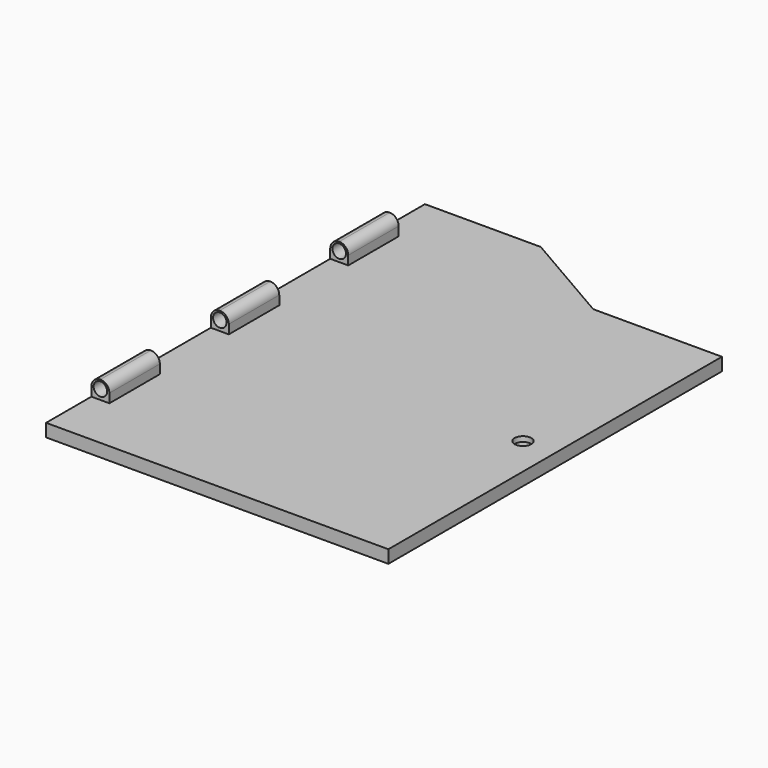
from build123d import *

# Parameters (mm, degrees)
F0_W     = 7
F0_H     = 24.5
F1_DEPTH = 5
F2_W     = 7
F2_H     = 24.5
F3_DEPTH = 7
F4_R     = 3.49999
F5_R     = 2.625
F6_DEPTH = 162.001
F7_R     = 3.25
F8_DEPTH = 2


# Not quite as in the source:
# - a fillet or chamfer is up to 0.001 mm smaller than in the source, because OpenCascade refuses the exact size


with BuildPart() as f1:
    # F0 (on Top) → F1 (new body)
    with BuildSketch(Plane.XY):
        Polygon((-34.0007612563, 142.7090217992), (-79.0007612563, 142.7090217992), (-79.0007612563, 121.2090217992), (-72.0007612563, 121.2090217992), (-72.0007612563, 96.7090217992), (-79.0007612563, 96.7090217992), (-79.0007612563, 63.2090217992), (-72.0007612563, 63.2090217992), (-72.0007612563, 38.7090217992), (-79.0007612563, 38.7090217992), (-79.0007612563, 5.2090217992), (-72.0007612563, 5.2090217992), (-72.0007612563, -19.2909782008), (-79.0007612563, -19.2909782008), (-79.0007612563, -41.2909782008), (53.9992387437, -41.2909782008), (53.9992387437, 120.7090218186), (3.9992387437, 120.7090218186), align=None)
        with Locations((-75.5007612563, 108.9590217992)):
            Rectangle(F0_W, F0_H)
        with Locations((-75.5007612563, 50.9590217992)):
            Rectangle(F0_W, F0_H)
        with Locations((-75.5007612563, -7.0409782008)):
            Rectangle(F0_W, F0_H)
    extrude(amount=F1_DEPTH)

    # F2 (on face) → F3 (join)
    with BuildSketch(Plane.XY.offset(5)):
        with Locations((-75.5007612563, 108.9590217992)):
            Rectangle(F2_W, F2_H)
        with Locations((-75.5007612563, 50.9590217992)):
            Rectangle(F2_W, F2_H)
        with Locations((-75.5007612563, -7.0409782008)):
            Rectangle(F2_W, F2_H)
    extrude(amount=F3_DEPTH)

    # F4 (radius 3.5 in the source; OpenCascade refuses exactly that, so slightly less here)
    f4_edges = [f1.edges().sort_by_distance(p)[0] for p in [
        (-72.000761, 108.959022, 12),
        (-72.000761, 50.959022, 12),
        (-79.000761, 50.959022, 12),
        (-79.000761, 108.959022, 12),
        (-72.000761, -7.040978, 12),
        (-79.000761, -7.040978, 12),
    ]]
    fillet(f4_edges, radius=F4_R)

    # F5 (on face) → F6 (cut, through all)
    with BuildSketch(Plane.XZ.offset(19.2909782008)):
        with Locations((-75.5007612563, 8.75)):
            Circle(F5_R)
    extrude(amount=-F6_DEPTH, mode=Mode.SUBTRACT)

    # F7 (on face) → F8 (cut)
    with BuildSketch(Plane.XY.offset(5)):
        with Locations((41.4992387437, 39.7090218089)):
            Circle(F7_R)
    extrude(amount=-F8_DEPTH, mode=Mode.SUBTRACT)


solid = f1.part
